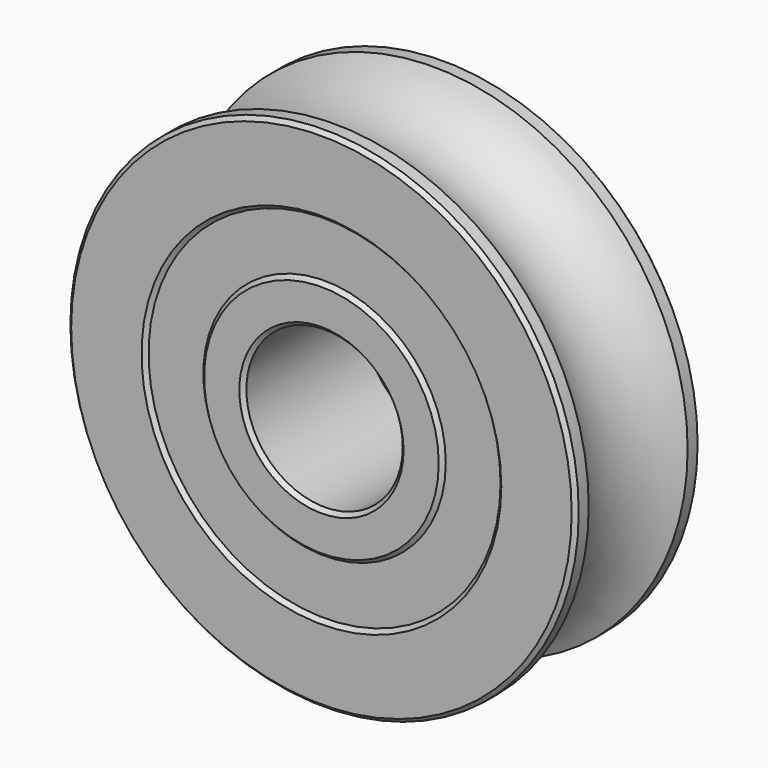
from build123d import *

# Parameters (mm, degrees)
F0_R     = 4.5
F0_R_2   = 3
F1_DEPTH = 1.9
F0_R_3   = 6.5
F0_R_4   = 2
F2_DEPTH = 2
F3_R     = 1.75
F5_SIZE  = 0.09999


# Not quite as in the source:
# - a fillet or chamfer is up to 0.001 mm smaller than in the source, because OpenCascade refuses the exact size


with BuildPart() as f1:
    # F0 (on Front) → F1 (new body, symmetric)
    with BuildSketch(Plane.XZ):
        Circle(F0_R)
        Circle(F0_R_2, mode=Mode.SUBTRACT)
    extrude(amount=F1_DEPTH, both=True)

    # F0 (on Front) → F2 (join, symmetric)
    with BuildSketch(Plane.XZ):
        Circle(F0_R_3)
        Circle(F0_R, mode=Mode.SUBTRACT)
        Circle(F0_R_2)
        Circle(F0_R_4, mode=Mode.SUBTRACT)
    extrude(amount=F2_DEPTH, both=True)

    # F4: sweep along a path in F4_path
    with BuildLine(Plane(origin=(6.5, -2, 0), x_dir=(0, 0, -1), z_dir=(0, 1, 0))) as f4_path:
        CenterArc((0, 6.5), 6.5, 0, 360)
    # F3 (on Right) → F4 (sweep, cut)
    with BuildSketch(Plane.YZ):
        with Locations((0, 7.25)):
            Circle(F3_R)
    sweep(path=f4_path.line, mode=Mode.SUBTRACT)

    # F5 (size 0.1 in the source; OpenCascade refuses exactly that, so slightly less here)
    f5_edges = [f1.edges().sort_by_distance(p)[0] for p in [
        (-6.5, -2, 0),
        (-4.5, -2, 0),
        (-3, -1.9, 0),
        (-2, -2, 0),
        (-2, 2, 0),
        (-3, 2, 0),
        (-4.5, 2, 0),
        (-6.5, 2, 0),
    ]]
    chamfer(f5_edges, length=F5_SIZE)


solid = f1.part
